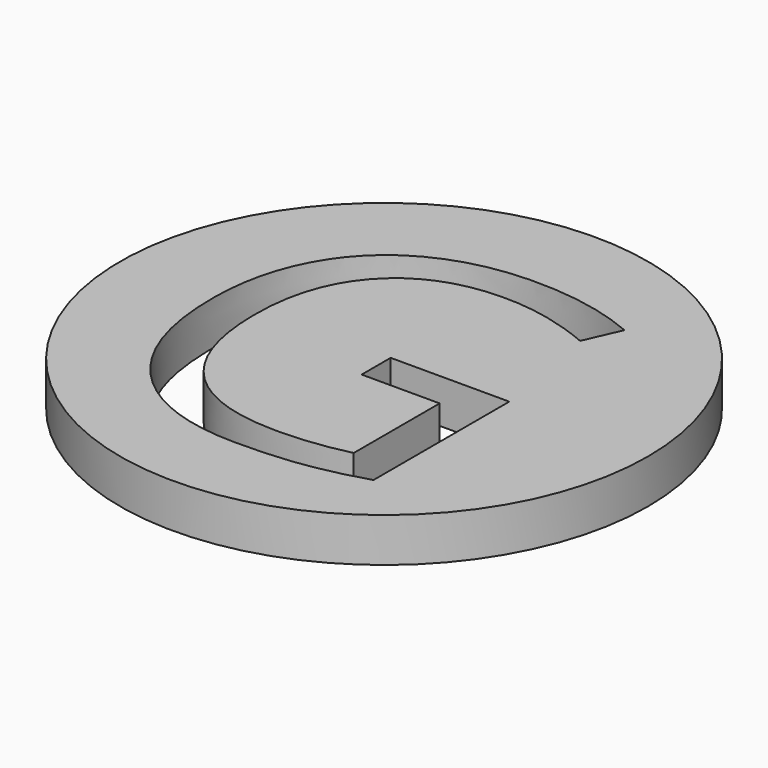
from build123d import *

# Parameters (mm, degrees)
F0_R         = 12
F1_DEPTH     = 2
F2_TEXT_SIZE = 22.2222222222
F3_DEPTH     = 25


# Not quite as in the source:
# - Text() gives the source's letters only with a copy of the font that has no kerning and outlines rounded to 1/6400 em; it was checked with that copy


with BuildPart() as f1:
    # F0 (on Top) → F1 (new body)
    with BuildSketch(Plane.XY):
        Circle(F0_R)
    extrude(amount=F1_DEPTH)

    # F2 (on face) → F3 (cut)
    with BuildSketch(Plane.XY.offset(2)):
        with Locations((-9.0322569013, -8.0967752114)):
            Text('G', F2_TEXT_SIZE, font='Open Sans', text_align=(TextAlign.LEFT, TextAlign.BOTTOM))
    extrude(amount=-F3_DEPTH, mode=Mode.SUBTRACT)


solid = f1.part
